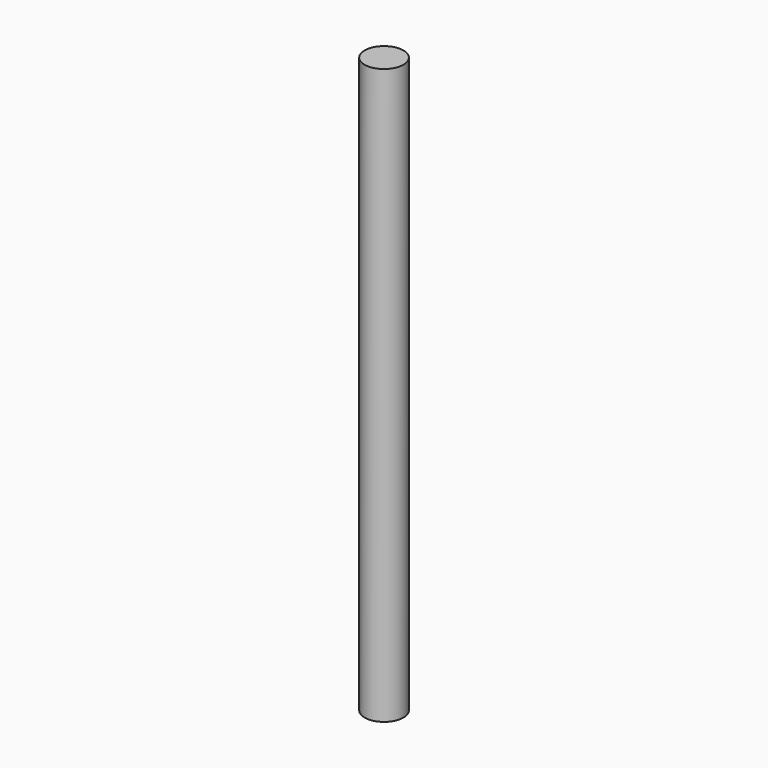
from build123d import *

# Parameters (mm, degrees)
F0_R     = 29.1786501147
F2_DEPTH = 863.6


# Not quite as in the source:
# - the program builds the solid bodies; features that only make, move or delete a surface that nothing else refers to are left out


with BuildPart() as f2:
    # F0 (on Top) → F2 (new body)
    with BuildSketch(Plane.XY):
        Circle(F0_R)
    extrude(amount=-F2_DEPTH)


solid = f2.part
